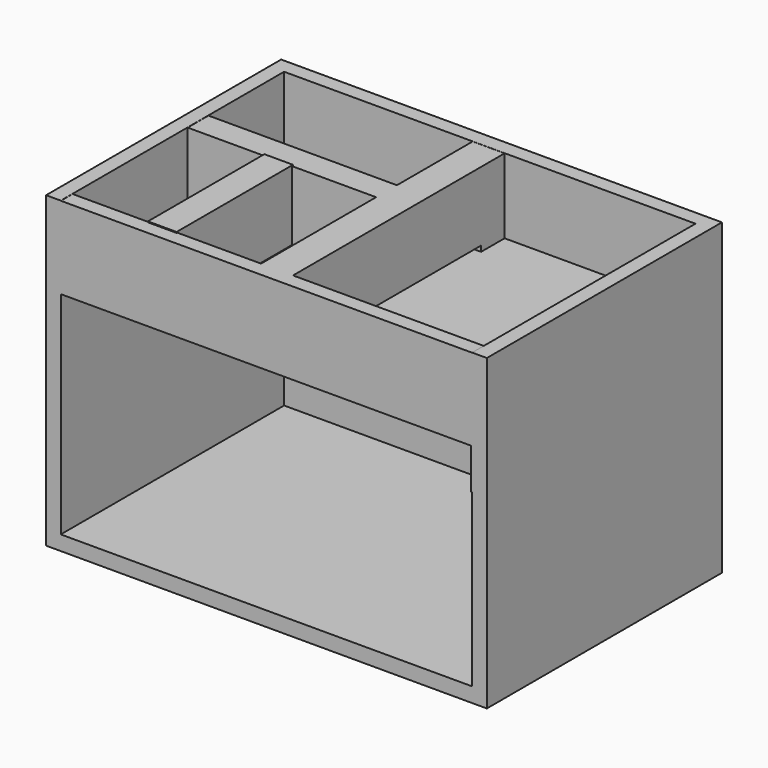
from build123d import *

# Parameters (mm, degrees)
F0_W      = 150
F0_H      = 100
F1_DEPTH  = 5
F2_W      = 5
F2_H      = 100
F3_DEPTH  = 100
F4_W      = 145
F4_H      = 5
F5_DEPTH  = 100
F6_W      = 5
F6_H      = 95
F7_DEPTH  = 100
F8_W      = 140
F8_H      = 5
F9_DEPTH  = 100
F10_W     = 140
F10_H     = 5
F11_DEPTH = 36.8
F12_W     = 10.8797177672
F12_H     = 90
F13_DEPTH = 36.8
F15_W     = 64.1449913383
F15_H     = 8.8397674263
F16_DEPTH = 36.8
F17_W     = 9.7464099526
F17_H     = 48.5053984448
F18_DEPTH = 37.1
F19_DEPTH = 1
F20_W     = 139.6295134723
F20_H     = 18.2434022427
F21_DEPTH = 85
F22_W     = 95
F22_H     = 2.5124400854
F23_DEPTH = 142.2
F25_DEPTH = 3


with BuildPart() as f1:
    # F0 (on Top) → F1 (new body)
    with BuildSketch(Plane.XY):
        with Locations((-36.598560214, 32.1514412761)):
            Rectangle(F0_W, F0_H)
    extrude(amount=F1_DEPTH)

    # F2 (on face) → F3 (join)
    with BuildSketch(Plane.XY.offset(5)):
        with Locations((-109.098560214, 32.1514412761)):
            Rectangle(F2_W, F2_H)
    extrude(amount=F3_DEPTH)

    # F4 (on face) → F5 (join)
    with BuildSketch(Plane.XY.offset(5)):
        with Locations((-34.098560214, 79.6514412761)):
            Rectangle(F4_W, F4_H)
    extrude(amount=F5_DEPTH)

    # F6 (on face) → F7 (join)
    with BuildSketch(Plane.XY.offset(5)):
        with Locations((35.901439786, 29.6514412761)):
            Rectangle(F6_W, F6_H)
    extrude(amount=F7_DEPTH)

    # F8 (on face) → F9 (join)
    with BuildSketch(Plane.XZ.offset(17.8485587239)):
        with Locations((-36.598560214, 65.6586462259)):
            Rectangle(F8_W, F8_H)
    extrude(amount=-F9_DEPTH)

    # F10 (on face) → F11 (join)
    with BuildSketch(Plane.XY.offset(68.1586462259)):
        with Locations((-36.598560214, -15.3485587239)):
            Rectangle(F10_W, F10_H)
    extrude(amount=F11_DEPTH)

    # F12 (on face) → F13 (join)
    with BuildSketch(Plane.XY.offset(68.1586462259)):
        with Locations((-36.9987897575, 32.1514412761)):
            Rectangle(F12_W, F12_H)
    extrude(amount=F13_DEPTH)

    # F15 (on face) → F16 (join)
    with BuildSketch(Plane.XY.offset(68.1586462259)):
        with Locations((-74.5111443102, 40.5214224011)):
            Rectangle(F15_W, F15_H)
    extrude(amount=F16_DEPTH)

    # F17 (on face) → F18 (join)
    with BuildSketch(Plane.XY.offset(68.1586462259)):
        with Locations((-75.8711062372, 11.1688547768)):
            Rectangle(F17_W, F17_H)
    extrude(amount=F18_DEPTH)

    # F19 (add): a face of the model
    f19_faces = [f1.faces().sort_by_distance(p)[0] for p in [
        (-75.8711062372, 35.4215539992, 86.7086462259),
    ]]
    extrude(f19_faces, amount=F19_DEPTH)

    # F20 (on face) → F21 (cut)
    with BuildSketch(Plane.XZ.offset(17.8485587239)):
        with Locations((-36.7838034779, 72.2803473473)):
            Rectangle(F20_W, F20_H)
    extrude(amount=-F21_DEPTH, mode=Mode.SUBTRACT)

    # F22 (on face) → F23 (join)
    with BuildSketch(Plane.YZ.offset(-106.598560214)):
        with Locations((29.6514412761, 78.2460346818)):
            Rectangle(F22_W, F22_H)
    extrude(amount=F23_DEPTH)

    # F24 (on face) → F25 (join)
    with BuildSketch(Plane(origin=(0, 0, 81.4020484686), x_dir=(1, 0, 0), z_dir=(0, 0, -1))):
        Polygon((33.0309532583, 17.8485587239), (-106.598560214, 17.8485587239), (-106.598560214, 12.8485587239), (-80.7443112135, 12.8485587239), (-70.9979012609, 12.8485587239), (-42.4386486411, 12.8485587239), (-31.5589308739, 12.8485587239), (33.0309532583, 12.8485587239), align=None)
    extrude(amount=F25_DEPTH)


solid = f1.part
